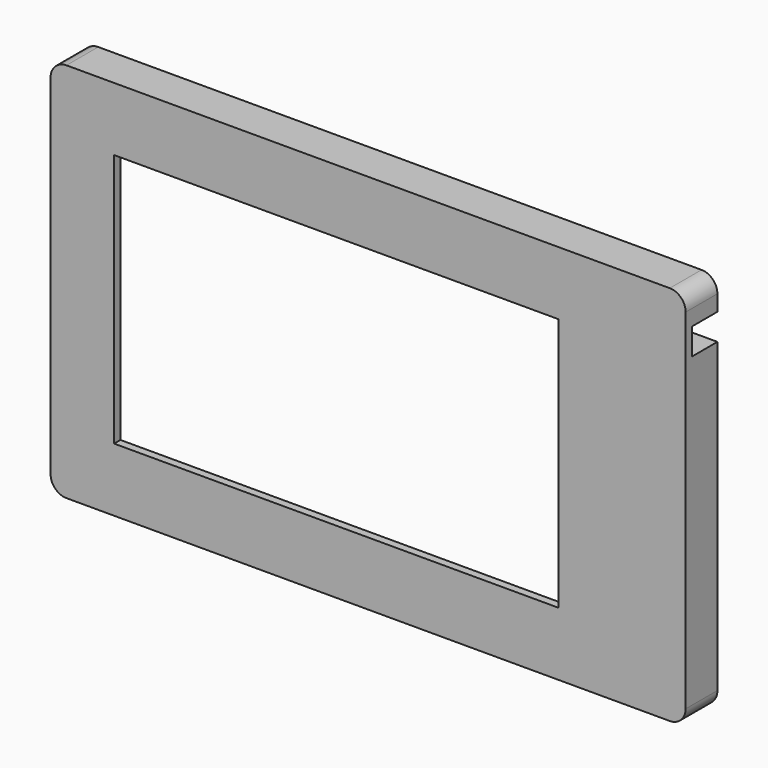
from build123d import *

# Parameters (mm, degrees)
F1_DEPTH      = 12.7
F2_W          = 508
F2_H          = 304.8
F2_W_2        = 355.6
F2_H_2        = 203.2
F3_DEPTH      = 6.35
F4_R          = 12.7
F5_W          = 76.2
F5_H          = 25.4
F6_DEPTH      = 3.81
F6_DEPTH_BACK = 25.4
F8_DEPTH      = 87.376
F9_W          = 63.5
F9_H          = 25.4
F10_DEPTH     = 3.81
F12_DEPTH     = 76.2


with BuildPart() as f1:
    # F0 (on Front) → F1 (new body, symmetric)
    with BuildSketch(Plane.XZ):
        Polygon((254, -17.3418857157), (203.2, -17.3418857157), (203.2, -127), (-203.2, -127), (-203.2, 127), (203.2, 127), (203.2, 14.4019788131), (241.3, 14.4019788131), (241.3, 127), (279.4, 127), (279.4, 152.4), (254, 152.4), (241.3, 152.4), (-228.6, 152.4), (-228.6, -152.4), (279.4, -152.4), (279.4, 105.8309227228), (254, 105.8309227228), (254, 0), align=None)
    extrude(amount=F1_DEPTH, both=True)

    # F2 (on face) → F3 (join)
    with BuildSketch(Plane.XZ.offset(12.7)):
        with Locations((25.4, 0)):
            Rectangle(F2_W, F2_H)
        Rectangle(F2_W_2, F2_H_2, mode=Mode.SUBTRACT)
    extrude(amount=F3_DEPTH)

    # F4
    f4_edges = [f1.edges().sort_by_distance(p)[0] for p in [
        (279.4, -3.175, -152.4),
        (-228.6, -3.175, -152.4),
        (-228.6, -3.175, 152.4),
        (279.4, -3.175, 152.4),
    ]]
    fillet(f4_edges, radius=F4_R)

    # F5 (on face) → F6 (join, two sides)
    with BuildSketch(Plane.XY.offset(-127)) as f6_sk:
        with Locations((-114.3, 0)):
            Rectangle(F5_W, F5_H)
    extrude(amount=F6_DEPTH)
    extrude(f6_sk.sketch, amount=-F6_DEPTH_BACK)

    # F7 (on face) → F8 (cut)
    with BuildSketch(Plane.YZ.offset(-76.2)):
        with BuildLine():
            add(Edge.make_bspline(
                [(12.7, -123.19), (10.5594976368, -123.19), (10.9031747427, -126.1164686911), (10.1332584811, -126.8581633475), (6.7809096129, -127)],
                knots=[0, 0, 0, 0, 0.2592828913, 0.6394583018, 0.6394583018, 0.6394583018, 0.6394583018], degree=3))
            Line((12.7, -123.19), (-12.7, -123.19))
            Line((-12.7, -123.19), (-12.7, -127))
            Line((-12.7, -127), (6.7809096129, -127))
        make_face()
    extrude(amount=-F8_DEPTH, mode=Mode.SUBTRACT)

    # F9 (on face) → F10 (join)
    with BuildSketch(Plane(origin=(0, 0, 127), x_dir=(1, 0, 0), z_dir=(0, 0, -1))):
        with Locations((120.65, 0)):
            Rectangle(F9_W, F9_H)
    extrude(amount=F10_DEPTH)

    # F11 (on face) → F12 (cut)
    with BuildSketch(Plane.YZ.offset(152.4)):
        with BuildLine():
            Line((-12.7, 123.19), (12.7, 123.19))
            add(Edge.make_bspline(
                [(12.7, 123.19), (10.4529513046, 123.19), (11.7430118211, 126.146945185), (9.7733114077, 126.8663682916), (5.5950677895, 127)],
                knots=[0, 0, 0, 0, 0.2484068186, 0.6533950313, 0.6533950313, 0.6533950313, 0.6533950313], degree=3))
            Line((5.5950677895, 127), (-12.7, 127))
            Line((-12.7, 127), (-12.7, 123.19))
        make_face()
    extrude(amount=-F12_DEPTH, mode=Mode.SUBTRACT)


solid = f1.part
